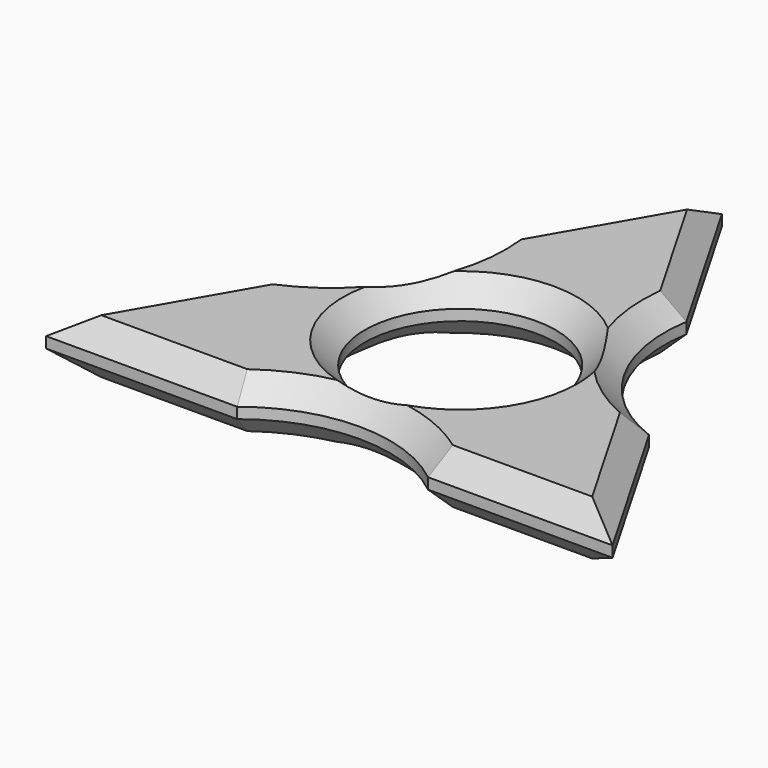
from build123d import *

# Parameters (mm, degrees)
F0_R          = 38.1
F0_R_2        = 11.1125
F1_DEPTH      = 3.175
F1_DEPTH_BACK = 3.175
F3_DEPTH      = 25.4
F5_DEPTH      = 25.4
F6_T1_DEPTH   = 34.5170750052
F6_T3_DEPTH   = 35.0734141938
F6_T5_DEPTH   = 34.5549539208
F6_T7_DEPTH   = 35.3294952256
F6_T9_DEPTH   = 35.0734141938
F6_T11_DEPTH  = 34.5170750052
F6_T14_ANGLE  = 120.7671426779
F6_T16_ANGLE  = 119.4565466951
F6_T18_ANGLE  = 120.7671426779
F6_T22_ANGLE  = 120.7671426779
F6_T24_ANGLE  = 119.4565466951
F6_T26_ANGLE  = 120.7671426779


# Not quite as in the source:
# - a fillet or chamfer that OpenCascade refuses, or shapes differently, is made with other operations: its cross-section is extruded or revolved along the edge and cut away or added


with BuildPart() as f1:
    # F0 (on Top) → F1 (new body, two sides)
    with BuildSketch(Plane.XY) as f1_sk:
        Circle(F0_R)
        Circle(F0_R_2, mode=Mode.SUBTRACT)
    extrude(amount=F1_DEPTH)
    extrude(f1_sk.sketch, amount=-F1_DEPTH_BACK)

    # F2 (on face) → F3 (cut)
    with BuildSketch(Plane.XY.offset(3.175)):
        with BuildLine():
            Line((-32.9882322762, -19.0627), (0, 38.1))
            ThreePointArc((0, 38.1), (-32.9992338547, 19.0436489413), (-32.9882322762, -19.0627))
        make_face()
        with BuildLine():
            Line((32.9882322762, -19.0627), (-32.9882322762, -19.0627))
            ThreePointArc((-32.9882322762, -19.0627), (0, -38.1), (32.9882322762, -19.0627))
        make_face()
        with BuildLine():
            ThreePointArc((38.1, 0), (26.9407683632, 26.9407683632), (0, 38.1))
            Line((0, 38.1), (32.9882322762, -19.0627))
            ThreePointArc((32.9882322762, -19.0627), (36.7998753376, -9.8680887277), (38.1, 0))
        make_face()
    extrude(amount=-F3_DEPTH, mode=Mode.SUBTRACT)

    # F4 (on face) → F5 (cut)
    with BuildSketch(Plane.XY.offset(3.175)):
        with BuildLine():
            Line((-10.7228866295, 19.5191574013), (-21.9872687911, 0))
            ThreePointArc((-21.9872687911, 0), (-12.8675975863, 7.7469760001), (-10.7228866295, 19.5191574013))
        make_face()
        with BuildLine():
            Line((21.9872687911, 0), (10.7228866295, 19.5191574013))
            ThreePointArc((10.7228866295, 19.5191574013), (12.8675975863, 7.7469760001), (21.9872687911, 0))
        make_face()
        with BuildLine():
            ThreePointArc((11.4974279343, -19.0627), (0.3872706524, -15.1640834027), (-10.7228866295, -19.0627))
            Line((-10.7228866295, -19.0627), (11.4974279343, -19.0627))
        make_face()
    extrude(amount=-F5_DEPTH, mode=Mode.SUBTRACT)

    # F6: chamfer of 2.54 on 20 edges, made by hand

    # F6_s2 → F6_t1 (cut)
    with BuildSketch(Plane(origin=(-19.7590646722, 34.2389212213, 0), x_dir=(0, 0, 1), z_dir=(0.4998333055, -0.8661216235, 0))):
        Polygon((3.175, -16.5036489413), (0.635, -19.0436489413), (3.175, -19.0436489413), align=None)
        Polygon((-3.175, -16.5036489413), (-0.635, -19.0436489413), (-3.175, -19.0436489413), align=None)
    extrude(amount=F6_T1_DEPTH, mode=Mode.SUBTRACT)

    # F6_s4 → F6_t3 (cut)
    with BuildSketch(Plane(origin=(2.2282041189, -3.8610787787, 0), x_dir=(0, 0, 1), z_dir=(0.4998333055, -0.8661216235, 0))):
        Polygon((3.175, -16.5036489413), (0.635, -19.0436489413), (3.175, -19.0436489413), align=None)
        Polygon((-3.175, -16.5036489413), (-0.635, -19.0436489413), (-3.175, -19.0436489413), align=None)
    extrude(amount=F6_T3_DEPTH, mode=Mode.SUBTRACT)

    # F6_s6 → F6_t5 (cut)
    with BuildSketch(Plane.YZ.offset(4.9653531448)):
        Polygon((-16.5227, 3.175), (-19.0627, 0.635), (-19.0627, 3.175), align=None)
        Polygon((-16.5227, -3.175), (-19.0627, -0.635), (-19.0627, -3.175), align=None)
    extrude(amount=F6_T5_DEPTH, mode=Mode.SUBTRACT)

    # F6_s8 → F6_t7 (cut)
    with BuildSketch(Plane.YZ.offset(-39.5203070657)):
        Polygon((-16.5227, 3.175), (-19.0627, 0.635), (-19.0627, 3.175), align=None)
        Polygon((-16.5227, -3.175), (-19.0627, -0.635), (-19.0627, -3.175), align=None)
    extrude(amount=F6_T7_DEPTH, mode=Mode.SUBTRACT)

    # F6_s10 → F6_t9 (cut)
    with BuildSketch(Plane(origin=(-19.7590646722, -34.2389212213, 0), x_dir=(0, 0, 1), z_dir=(0.4998333055, 0.8661216235, 0))):
        Polygon((0.635, -19.0436489413), (3.175, -16.5036489413), (3.175, -19.0436489413), align=None)
        Polygon((-0.635, -19.0436489413), (-3.175, -16.5036489413), (-3.175, -19.0436489413), align=None)
    extrude(amount=F6_T9_DEPTH, mode=Mode.SUBTRACT)

    # F6_s12 → F6_t11 (cut)
    with BuildSketch(Plane(origin=(2.5062809746, 4.3429361799, 0), x_dir=(0, 0, 1), z_dir=(0.4998333055, 0.8661216235, 0))):
        Polygon((3.175, -16.5036489413), (0.635, -19.0436489413), (3.175, -19.0436489413), align=None)
        Polygon((-3.175, -16.5036489413), (-0.635, -19.0436489413), (-3.175, -19.0436489413), align=None)
    extrude(amount=F6_T11_DEPTH, mode=Mode.SUBTRACT)

    # F6_s13 → F6_t14 (revolve, cut)
    with BuildSketch(Plane(origin=(14.4954043102, 24.71215529, 0), x_dir=(0, 0, 1), z_dir=(0.505952459, 0.8625613655, 0))):
        Polygon((3.175, -4.353790183), (0.635, -1.813790183), (3.175, -1.813790183), align=None)
    revolve(axis=Axis((28.2672400519, 16.6340121728, 3.175), (0, 0, 1)), revolution_arc=F6_T14_ANGLE, mode=Mode.SUBTRACT)

    # F6_s15 → F6_t16 (revolve, cut)
    with BuildSketch(Plane(origin=(14.4410953434, -24.7409917864, 0), x_dir=(0, 0, 1), z_dir=(0.5041015086, -0.8636444112, 0))):
        Polygon((3.175, -4.0473019905), (0.635, -1.5073019905), (3.175, -1.5073019905), align=None)
    revolve(axis=Axis((0.3872706524, -32.9440834027, 3.175), (0, 0, 1)), revolution_arc=F6_T16_ANGLE, mode=Mode.SUBTRACT)

    # F6_s17 → F6_t18 (revolve, cut)
    with BuildSketch(Plane(origin=(-28.374198152, 0.1844947944, 0), x_dir=(0, 0, 1), z_dir=(-0.9999788613, 0.0065020655, 0))):
        Polygon((3.175, -3.8701348937), (0.635, -1.3301348937), (3.175, -1.3301348937), align=None)
    revolve(axis=Axis((-28.2672400519, 16.6340121728, 3.175), (0, 0, 1)), revolution_arc=F6_T18_ANGLE, mode=Mode.SUBTRACT)

    # F6_s19 → F6_t20 (revolve, cut)
    with BuildSketch(Plane.XZ):
        Polygon((13.6525, 3.175), (11.1125, 0.635), (11.1125, 3.175), align=None)
    revolve(axis=Axis((0, 0, 3.175), (0, 0, 1)), mode=Mode.SUBTRACT)

    # F6_s21 → F6_t22 (revolve, cut)
    with BuildSketch(Plane(origin=(14.4954043102, 24.71215529, 0), x_dir=(0, 0, 1), z_dir=(0.505952459, 0.8625613655, 0))):
        Polygon((-3.175, -4.353790183), (-0.635, -1.813790183), (-3.175, -1.813790183), align=None)
    revolve(axis=Axis((28.2672400519, 16.6340121728, -3.175), (0, 0, 1)), revolution_arc=F6_T22_ANGLE, mode=Mode.SUBTRACT)

    # F6_s23 → F6_t24 (revolve, cut)
    with BuildSketch(Plane(origin=(14.4410953434, -24.7409917864, 0), x_dir=(0, 0, 1), z_dir=(0.5041015086, -0.8636444112, 0))):
        Polygon((-3.175, -4.0473019905), (-0.635, -1.5073019905), (-3.175, -1.5073019905), align=None)
    revolve(axis=Axis((0.3872706524, -32.9440834027, -3.175), (0, 0, 1)), revolution_arc=F6_T24_ANGLE, mode=Mode.SUBTRACT)

    # F6_s25 → F6_t26 (revolve, cut)
    with BuildSketch(Plane(origin=(-28.374198152, 0.1844947944, 0), x_dir=(0, 0, 1), z_dir=(-0.9999788613, 0.0065020655, 0))):
        Polygon((-0.635, -1.3301348937), (-3.175, -3.8701348937), (-3.175, -1.3301348937), align=None)
    revolve(axis=Axis((-28.2672400519, 16.6340121728, -3.175), (0, 0, 1)), revolution_arc=F6_T26_ANGLE, mode=Mode.SUBTRACT)

    # F6_s27 → F6_t28 (revolve, cut)
    with BuildSketch(Plane.XZ):
        Polygon((13.6525, -3.175), (11.1125, -0.635), (11.1125, -3.175), align=None)
    revolve(axis=Axis((0, 0, -3.175), (0, 0, 1)), mode=Mode.SUBTRACT)


solid = f1.part
